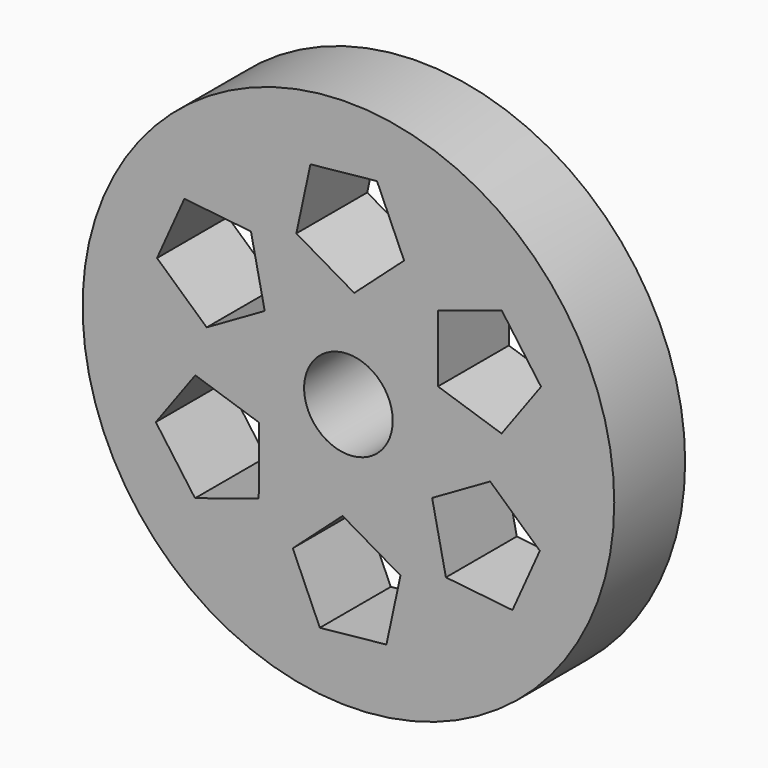
from build123d import *

# Parameters (mm, degrees)
F0_R            = 38.1
F1_DEPTH        = 12.7
F2_R            = 6.35
F3_DEPTH        = 12.701
F5_DEPTH        = 12.701
F5_COPIES_COUNT = 6


# Not quite as in the source:
# - a pattern or mirror of a feature is missing from the dataset's text; its kind, count and spacing are read off the source's solid


with BuildPart() as f1:
    # F0 (on Front) → F1 (new body)
    with BuildSketch(Plane.XZ):
        Circle(F0_R)
    extrude(amount=F1_DEPTH)

    # F2 (on face) → F3 (cut, through all)
    with BuildSketch(Plane.XZ.offset(12.7)):
        Circle(F2_R)
    extrude(amount=-F3_DEPTH, mode=Mode.SUBTRACT)

    # F4 (on face) → F5 (cut, through all)
    with BuildSketch(Plane.XZ.offset(12.7)):
        Polygon((0.8353452235, 14.3352959198), (7.9783069864, 20.7387890774), (4.0955196667, 29.5109376166), (-5.4471366308, 28.5289304107), (-7.4620352459, 19.149868041), align=None)
    f5 = extrude(amount=-F5_DEPTH, mode=Mode.SUBTRACT)

    # F5_copies: F5 ×6 about axis
    f5_copies_axis = Axis((0, 0, 0), (0, 1, 0))
    for i in range(1, F5_COPIES_COUNT):
        add(f5.rotate(f5_copies_axis, i * 360 / F5_COPIES_COUNT), mode=Mode.SUBTRACT)


solid = f1.part
